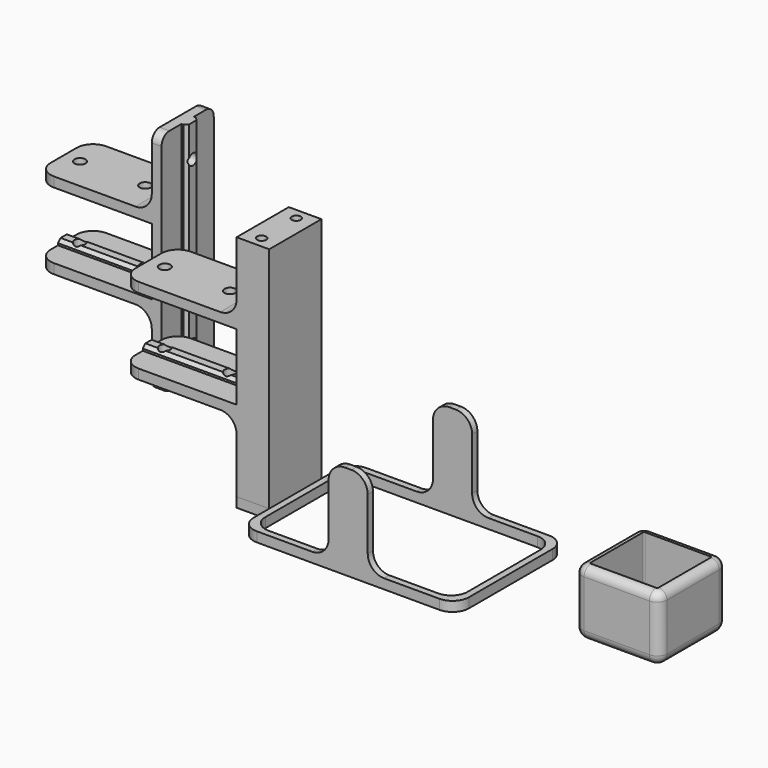
from build123d import *

# Parameters (mm, degrees)
F0_W         = 254
F0_H         = 508
F0_R         = 43.18
F1_DEPTH     = 76.2
F0_W_2       = 304.8
F0_H_2       = 50.8
F2_DEPTH     = 736.6
F3_R         = 127
F4_W         = 254
F4_H         = 508
F4_R         = 43.18
F4_R_2       = 35.56
F5_DEPTH     = 1778
F6_DEPTH     = 508
F7_R         = 35.56
F8_DEPTH     = 508
F9_W         = 508
F9_H         = 76.2
F10_DEPTH    = 889
F11_R        = 127
F12_R        = 43.18
F13_DEPTH    = 1300.481
F14_W        = 889
F14_H        = 111.76
F14_R        = 43.18
F15_DEPTH    = 40.64
F16_T1_DEPTH = 954.3207478943
F18_DEPTH    = 177.8
F19_R        = 76.2
F20_W        = 121.92
F20_H        = 1778
F20_R        = 43.18
F21_DEPTH    = 40.64
F22_T1_DEPTH = 1908.6414957887
F23_DEPTH    = 965.201
F25_DEPTH    = 508
F26_T        = -66.04
F27_R        = 43.18
F28_DEPTH    = 508.001
F29_R        = 76.2
F30_R        = 63.5


# Not quite as in the source:
# - a fillet or chamfer that OpenCascade refuses, or shapes differently, is made with other operations: its cross-section is extruded or revolved along the edge and cut away or added


with BuildPart() as f1:
    # F0 (on Top) → F1 (new body)
    with BuildSketch(Plane.XY):
        with Locations((-780.9189300537, 96.6712751389)):
            Rectangle(F0_W, F0_H)
        with Locations((-780.9189300537, -72.9987174273)):
            Circle(F0_R, mode=Mode.SUBTRACT)
        with Locations((-780.9189300537, 265.5358910561)):
            Circle(F0_R, mode=Mode.SUBTRACT)
        with BuildLine():
            ThreePointArc((-603.1189300537, 452.2712751389), (-565.9214912644, 542.0738363495), (-476.1189300537, 579.2712751389))
            Line((-476.1189300537, 579.2712751389), (31.8810699463, 579.2712751389))
            Line((31.8810699463, 579.2712751389), (31.8810699463, 630.0712751389))
            Line((31.8810699463, 630.0712751389), (-526.9189300537, 630.0712751389))
            ThreePointArc((-526.9189300537, 630.0712751389), (-616.7214912644, 592.8738363495), (-653.9189300537, 503.0712751389))
            Line((-653.9189300537, 503.0712751389), (-653.9189300537, 350.6712751389))
            Line((-653.9189300537, 350.6712751389), (-653.9189300537, -157.3287248611))
            Line((-653.9189300537, -157.3287248611), (-653.9189300537, -309.7287248611))
            ThreePointArc((-653.9189300537, -309.7287248611), (-616.7214912644, -399.5312860718), (-526.9189300537, -436.7287248611))
            Line((-526.9189300537, -436.7287248611), (31.8810699463, -436.7287248611))
            Line((31.8810699463, -436.7287248611), (31.8810699463, -385.9287248611))
            Line((31.8810699463, -385.9287248611), (-476.1189300537, -385.9287248611))
            ThreePointArc((-476.1189300537, -385.9287248611), (-565.9214912644, -348.7312860718), (-603.1189300537, -258.9287248611))
            Line((-603.1189300537, -258.9287248611), (-603.1189300537, 452.2712751389))
        make_face()
    extrude(amount=F1_DEPTH)



with BuildPart() as f1b:
    # F0 (on Top) → F1, piece 2 (new body)
    with BuildSketch(Plane.XY):
        with BuildLine():
            Line((336.6810699463, 630.0712751389), (336.6810699463, 579.2712751389))
            Line((336.6810699463, 579.2712751389), (844.6810699463, 579.2712751389))
            ThreePointArc((844.6810699463, 579.2712751389), (934.483631157, 542.0738363495), (971.6810699463, 452.2712751389))
            Line((971.6810699463, 452.2712751389), (971.6810699463, -258.9287248611))
            ThreePointArc((971.6810699463, -258.9287248611), (934.483631157, -348.7312860718), (844.6810699463, -385.9287248611))
            Line((844.6810699463, -385.9287248611), (336.6810699463, -385.9287248611))
            Line((336.6810699463, -385.9287248611), (336.6810699463, -436.7287248611))
            Line((336.6810699463, -436.7287248611), (895.4810699463, -436.7287248611))
            ThreePointArc((895.4810699463, -436.7287248611), (985.283631157, -399.5312860718), (1022.4810699463, -309.7287248611))
            Line((1022.4810699463, -309.7287248611), (1022.4810699463, 503.0712751389))
            ThreePointArc((1022.4810699463, 503.0712751389), (985.283631157, 592.8738363495), (895.4810699463, 630.0712751389))
            Line((895.4810699463, 630.0712751389), (336.6810699463, 630.0712751389))
        make_face()
    extrude(amount=F1_DEPTH)


with BuildPart() as f1_1:
    add(f1.part)

    add(f1b.part)  # F2 merges F1b
    # F0 (on Top) → F2 (join)
    with BuildSketch(Plane.XY):
        with Locations((184.2810699463, 604.6712751389)):
            Rectangle(F0_W_2, F0_H_2)
        with Locations((184.2810699463, -411.3287248611)):
            Rectangle(F0_W_2, F0_H_2)
    extrude(amount=F2_DEPTH)

    # F3
    f3_edges = [f1_1.edges().sort_by_distance(p)[0] for p in [
        (31.88107, -411.328725, 736.6),
        (336.68107, -411.328725, 736.6),
        (336.68107, 604.671275, 736.6),
        (31.88107, 604.671275, 736.6),
        (31.88107, 604.671275, 76.2),
        (31.88107, -411.328725, 76.2),
        (336.68107, -411.328725, 76.2),
        (336.68107, 604.671275, 76.2),
    ]]
    fillet(f3_edges, radius=F3_R)


with BuildPart() as f5:
    # F4 (on face) → F5 (new body)
    with BuildSketch(Plane.XY.offset(76.2)):
        with Locations((-780.9189300537, 96.6712751389)):
            Rectangle(F4_W, F4_H)
        with Locations((-780.9189300537, -72.9987174273)):
            Circle(F4_R, mode=Mode.SUBTRACT)
        with Locations((-780.9189300537, 265.5358910561)):
            Circle(F4_R, mode=Mode.SUBTRACT)
        with Locations((-780.9189300537, -72.9987174273)):
            Circle(F4_R)
        with Locations((-780.9189300537, -72.9987174273)):
            Circle(F4_R_2, mode=Mode.SUBTRACT)
        with Locations((-780.9189300537, 265.5358910561)):
            Circle(F4_R)
        with Locations((-780.9189300537, 265.5358910561)):
            Circle(F4_R_2, mode=Mode.SUBTRACT)
        with Locations((-780.9189300537, 265.5358910561)):
            Circle(F4_R_2)
        with Locations((-780.9189300537, -72.9987174273)):
            Circle(F4_R_2)
    extrude(amount=F5_DEPTH)

    # F4 (on face) → F6 (cut)
    with BuildSketch(Plane.XY.offset(76.2)):
        with Locations((-780.9189300537, 265.5358910561)):
            Circle(F4_R_2)
        with Locations((-780.9189300537, -72.9987174273)):
            Circle(F4_R_2)
    extrude(amount=F6_DEPTH, mode=Mode.SUBTRACT)

    # F7 (on face) → F8 (cut)
    with BuildSketch(Plane.XY.offset(1854.2)):
        with Locations((-780.9189300537, 264.8776769638)):
            Circle(F7_R)
        with Locations((-780.9189300537, -72.1629709005)):
            Circle(F7_R)
    extrude(amount=-F8_DEPTH, mode=Mode.SUBTRACT)

    # F9 (on face) → F10 (join)
    with BuildSketch(Plane(origin=(-907.9189300537, 0, 0), x_dir=(0, -1, 0), z_dir=(-1, 0, 0))):
        with Locations((-96.6712751389, 668.02)):
            Rectangle(F9_W, F9_H)
        with Locations((-96.6712751389, 1262.38)):
            Rectangle(F9_W, F9_H)
    extrude(amount=F10_DEPTH)

    # F11
    f11_edges = [f5.edges().sort_by_distance(p)[0] for p in [
        (-907.91893, 96.671275, 629.92),
        (-907.91893, 96.671275, 1300.48),
        (-1796.91893, -157.328725, 668.02),
        (-1796.91893, -157.328725, 1262.38),
        (-1796.91893, 350.671275, 1262.38),
        (-1796.91893, 350.671275, 668.02),
    ]]
    fillet(f11_edges, radius=F11_R)

    # F12 (on face) → F13 (cut, through all)
    with BuildSketch(Plane.XY.offset(1300.48)):
        with Locations((-1669.9189300537, 96.6712751389)):
            Circle(F12_R)
        with Locations((-1161.9189300537, 96.6712751389)):
            Circle(F12_R)
    extrude(amount=-F13_DEPTH, mode=Mode.SUBTRACT)

    # F14 (on face) → F15 (join)
    with BuildSketch(Plane.XY.offset(706.12)):
        with Locations((-1352.4189300537, 96.6712751389)):
            Rectangle(F14_W, F14_H)
        with Locations((-1669.9189300537, 96.6712751389)):
            Circle(F14_R, mode=Mode.SUBTRACT)
        with Locations((-1161.9189300537, 96.6712751389)):
            Circle(F14_R, mode=Mode.SUBTRACT)
    extrude(amount=F15_DEPTH)

    # F16: chamfer of 25.4 on 2 edges, made by hand

    # F16_s2 → F16_t1 (cut)
    with BuildSketch(Plane.YZ.offset(-1862.239677948)):
        Polygon((40.7912751389, 721.36), (66.1912751389, 746.76), (40.7912751389, 746.76), align=None)
        Polygon((152.5512751389, 721.36), (127.1512751389, 746.76), (152.5512751389, 746.76), align=None)
    extrude(amount=F16_T1_DEPTH, mode=Mode.SUBTRACT)


with BuildPart() as f17_1:
    # F17: copy of F5
    add(f5.part.moved(Location((-1270, 762, 0))))

    # F18 (cut): a face of the model
    f18_faces = [f17_1.faces().sort_by_distance(p)[0] for p in [
        (-1923.9189300537, 858.6712751389, 965.2),
    ]]
    extrude(f18_faces, amount=-F18_DEPTH, mode=Mode.SUBTRACT)

    # F19
    f19_edges = [f17_1.edges().sort_by_distance(p)[0] for p in [
        (-2139.81893, 604.671275, 1854.2),
        (-2139.81893, 1112.671275, 1854.2),
        (-2139.81893, 604.671275, 76.2),
        (-2139.81893, 1112.671275, 76.2),
    ]]
    fillet(f19_edges, radius=F19_R)

    # F20 (on face) → F21 (join)
    with BuildSketch(Plane.YZ.offset(-2101.7189300537)):
        with Locations((858.6712751389, 965.2)):
            Rectangle(F20_W, F20_H)
        with Locations((858.6712751389, 330.2)):
            Circle(F20_R, mode=Mode.SUBTRACT)
        with Locations((858.6712751389, 1600.2)):
            Circle(F20_R, mode=Mode.SUBTRACT)
    extrude(amount=F21_DEPTH)

    # F22: chamfer of 25.4 on 2 edges, made by hand

    # F22_s2 → F22_t1 (cut)
    with BuildSketch(Plane.XY.offset(10.8792521057)):
        Polygon((-2061.0789300537, 894.2312751389), (-2086.4789300537, 919.6312751389), (-2061.0789300537, 919.6312751389), align=None)
        Polygon((-2086.4789300537, 797.7112751389), (-2061.0789300537, 823.1112751389), (-2061.0789300537, 797.7112751389), align=None)
    extrude(amount=F22_T1_DEPTH, mode=Mode.SUBTRACT)

    # F20 (on face) → F23 (cut, through all)
    with BuildSketch(Plane.YZ.offset(-2101.7189300537)):
        with Locations((858.6712751389, 1600.2)):
            Circle(F20_R)
        with Locations((858.6712751389, 330.2)):
            Circle(F20_R)
    extrude(amount=-F23_DEPTH, mode=Mode.SUBTRACT)


with BuildPart() as f25:
    # F24 (on face) → F25 (new body)
    with BuildSketch(Plane.XY):
        with BuildLine():
            Line((1843.8097154617, -214.8184916639), (2351.8097154617, -214.8184916639))
            ThreePointArc((2351.8097154617, -214.8184916639), (2405.6912521881, -192.5000283903), (2428.0097154617, -138.6184916639))
            Line((2428.0097154617, -138.6184916639), (2428.0097154617, 369.3815083361))
            ThreePointArc((2428.0097154617, 369.3815083361), (2405.6912521881, 423.2630450625), (2351.8097154617, 445.5815083361))
            Line((2351.8097154617, 445.5815083361), (1843.8097154617, 445.5815083361))
            ThreePointArc((1843.8097154617, 445.5815083361), (1789.9281787353, 423.2630450625), (1767.6097154617, 369.3815083361))
            Line((1767.6097154617, 369.3815083361), (1767.6097154617, -138.6184916639))
            ThreePointArc((1767.6097154617, -138.6184916639), (1789.9281787353, -192.5000283903), (1843.8097154617, -214.8184916639))
        make_face()
    extrude(amount=F25_DEPTH)

    # F26
    f26_openings = [f25.faces().sort_by_distance(p)[0] for p in [
        (2097.809715, 115.381508, 508),
    ]]
    offset(amount=F26_T, openings=f26_openings)

    # F27 (on face) → F28 (cut, through all)
    with BuildSketch(Plane.XY.offset(508)):
        with Locations((2097.8097154617, 115.3815083361)):
            Circle(F27_R)
    extrude(amount=-F28_DEPTH, mode=Mode.SUBTRACT)

    # F29
    f29_edges = [f25.edges().sort_by_distance(p)[0] for p in [
        (2097.809715, -214.818492, 0),
    ]]
    fillet(f29_edges, radius=F29_R)

    # F30
    f30_edges = [f25.edges().sort_by_distance(p)[0] for p in [
        (2097.809715, 445.581508, 508),
    ]]
    fillet(f30_edges, radius=F30_R)


solid = Compound([f1_1.part, f5.part, f17_1.part, f25.part])
